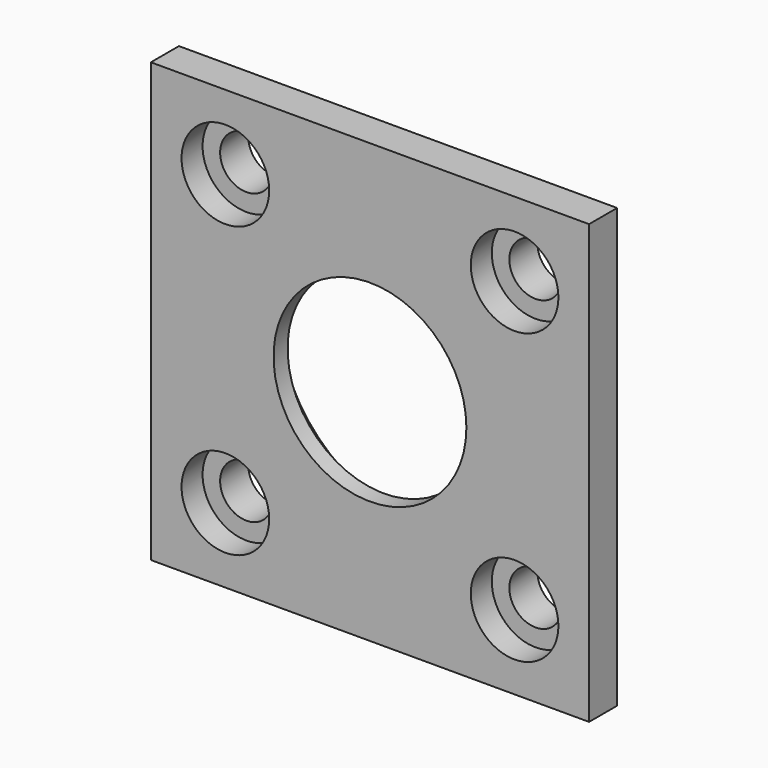
from build123d import *

# Parameters (mm, degrees)
F0_W      = 50
F0_H      = 50
F1_DEPTH  = 4
F2_W      = 43.4
F2_H      = 43.4
F3_DEPTH  = 3
F4_R      = 3
F5_DEPTH  = 25
F6_R      = 5
F6_R_2    = 3
F7_DEPTH  = 3
F8_R      = 16
F9_DEPTH  = 5
F10_R     = 11
F11_DEPTH = 25
F12_R     = 3


# Not quite as in the source:
# - a feature names something its author has since deleted; it is built from what else it names


with BuildPart() as f1:
    # F0 (on Front) → F1 (new body)
    with BuildSketch(Plane.XZ):
        Rectangle(F0_W, F0_H)
    extrude(amount=-F1_DEPTH)

    # F2 (on face) → F3 (join)
    with BuildSketch(Plane(origin=(0, 4, 0), x_dir=(-1, 0, 0), z_dir=(0, 1, 0))):
        Rectangle(F2_W, F2_H)
    extrude(amount=F3_DEPTH)

    # F4 (on face) → F5 (cut)
    with BuildSketch(Plane(origin=(0, 7, 0), x_dir=(-1, 0, 0), z_dir=(0, 1, 0))):
        with Locations((-16.5, 16.5)):
            Circle(F4_R)
        with Locations((16.5, 16.5)):
            Circle(F4_R)
        with Locations((16.5, -16.5)):
            Circle(F4_R)
        with Locations((-16.5, -16.5)):
            Circle(F4_R)
    extrude(amount=-F5_DEPTH, mode=Mode.SUBTRACT)

    # F6 (on face) → F7 (cut)
    with BuildSketch(Plane.XZ):
        with Locations((-16.5, 16.5)):
            Circle(F6_R)
        with Locations((-16.5, 16.5)):
            Circle(F6_R_2, mode=Mode.SUBTRACT)
        with Locations((16.5, 16.5)):
            Circle(F6_R)
        with Locations((16.5, 16.5)):
            Circle(F6_R_2, mode=Mode.SUBTRACT)
        with Locations((16.5, -16.5)):
            Circle(F6_R)
        with Locations((16.5, -16.5)):
            Circle(F6_R_2, mode=Mode.SUBTRACT)
        with Locations((-16.5, -16.5)):
            Circle(F6_R)
        with Locations((-16.5, -16.5)):
            Circle(F6_R_2, mode=Mode.SUBTRACT)
    extrude(amount=-F7_DEPTH, mode=Mode.SUBTRACT)

    # F8 (on face) → F9 (cut)
    with BuildSketch(Plane(origin=(0, 7, 0), x_dir=(-1, 0, 0), z_dir=(0, 1, 0))):
        Circle(F8_R)
    extrude(amount=-F9_DEPTH, mode=Mode.SUBTRACT)

    # F10 (on face) → F11 (cut)
    with BuildSketch(Plane.XZ):
        Circle(F10_R)
    extrude(amount=-F11_DEPTH, mode=Mode.SUBTRACT)

    # F12
    f12_edges = [f1.edges().sort_by_distance(p)[0] for p in [
        (21.7, 5.5, 21.7),
        (-21.7, 5.5, 21.7),
        (-21.7, 5.5, -21.7),
        (21.7, 5.5, -21.7),
    ]]
    fillet(f12_edges, radius=F12_R)


solid = f1.part
